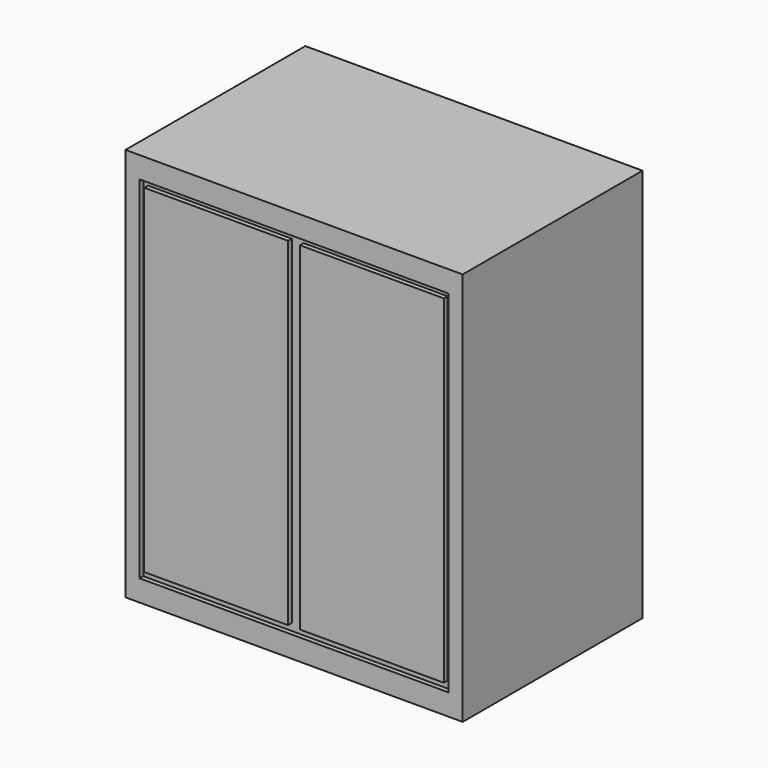
from build123d import *

# Parameters (mm, degrees)
F0_W     = 914.4
F0_H     = 1068.3875
F1_DEPTH = 304.8
F3_W     = 419.1
F3_H     = 952.5
F3_W_2   = 390.1610858738
F3_H_2   = 917.601108551
F5_DEPTH = 12.7


# Not quite as in the source:
# - the program builds the solid bodies; features that only make, move or delete a surface that nothing else refers to are left out


with BuildPart() as f1:
    # F0 (on Front) → F1 (new body, symmetric)
    with BuildSketch(Plane.XZ):
        with Locations((0, 534.19375)):
            Rectangle(F0_W, F0_H)
    extrude(amount=F1_DEPTH, both=True)

    # F3 (on face) → F5 (cut)
    with BuildSketch(Plane.XZ.offset(304.8)):
        with Locations((-209.55, 534.19375)):
            Rectangle(F3_W, F3_H)
        with Locations((-211.3307770342, 535.7740521431)):
            Rectangle(F3_W_2, F3_H_2, mode=Mode.SUBTRACT)
        with Locations((209.55, 534.19375)):
            Rectangle(F3_W, F3_H)
        with Locations((211.3307770342, 535.7740521431)):
            Rectangle(F3_W_2, F3_H_2, mode=Mode.SUBTRACT)
    extrude(amount=-F5_DEPTH, mode=Mode.SUBTRACT)


solid = f1.part
